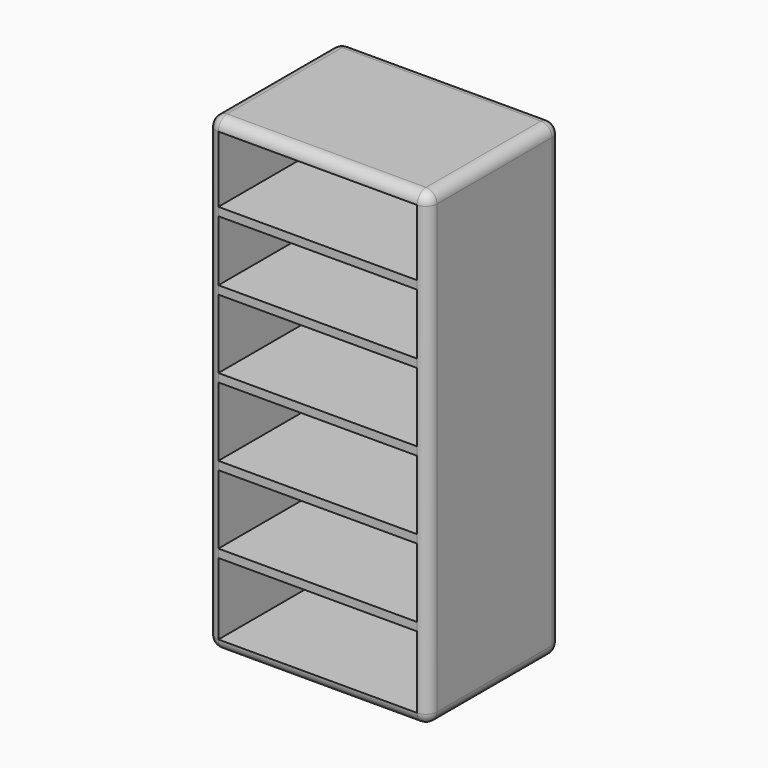
from build123d import *

# Parameters (mm, degrees)
F0_W      = 800
F0_H      = 1700
F1_DEPTH  = 600
F2_T      = -40
F3_W      = 720
F3_H      = 30
F4_DEPTH  = 560
F5_R      = 39.99999
F7_DEPTH  = 560
F8_W      = 720
F8_H      = 30
F9_DEPTH  = 560
F10_W     = 720
F10_H     = 30
F11_DEPTH = 560


# Not quite as in the source:
# - a fillet or chamfer is up to 0.001 mm smaller than in the source, because OpenCascade refuses the exact size


with BuildPart() as f1:
    # F0 (on Front) → F1 (new body)
    with BuildSketch(Plane.XZ):
        Rectangle(F0_W, F0_H)
    extrude(amount=F1_DEPTH)

    # F2
    f2_openings = [f1.faces().sort_by_distance(p)[0] for p in [
        (0, -600, 0),
    ]]
    offset(amount=F2_T, openings=f2_openings)

    # F3 (on face) → F4 (join)
    with BuildSketch(Plane.XZ.offset(40)):
        with Locations((0, -255)):
            Rectangle(F3_W, F3_H)
    extrude(amount=F4_DEPTH)

    # F5 (radius 40 in the source; OpenCascade refuses exactly that, so slightly less here)
    f5_edges = [f1.edges().sort_by_distance(p)[0] for p in [
        (-400, -600, 0),
        (-400, -300, 850),
        (0, -600, 850),
        (400, -300, 850),
        (0, 0, 850),
        (-400, 0, 0),
        (400, 0, 0),
        (0, 0, -850),
        (-400, -300, -850),
        (400, -300, -850),
        (0, -600, -850),
        (400, -600, 0),
    ]]
    fillet(f5_edges, radius=F5_R)

    # F6 (on face) → F7 (join)
    with BuildSketch(Plane.XZ.offset(40)):
        Polygon((360, 40), (-360, 40), (-360, 20.5096974969), (-360, 10), (360, 10), align=None)
    extrude(amount=F7_DEPTH)

    # F8 (on face) → F9 (join)
    with BuildSketch(Plane.XZ.offset(40)):
        with Locations((0, -535)):
            Rectangle(F8_W, F8_H)
    extrude(amount=F9_DEPTH)

    # F10 (on face) → F11 (join)
    with BuildSketch(Plane.XZ.offset(40)):
        with Locations((0, 305)):
            Rectangle(F10_W, F10_H)
        with Locations((0, 555)):
            Rectangle(F10_W, F10_H)
    extrude(amount=F11_DEPTH)


solid = f1.part
